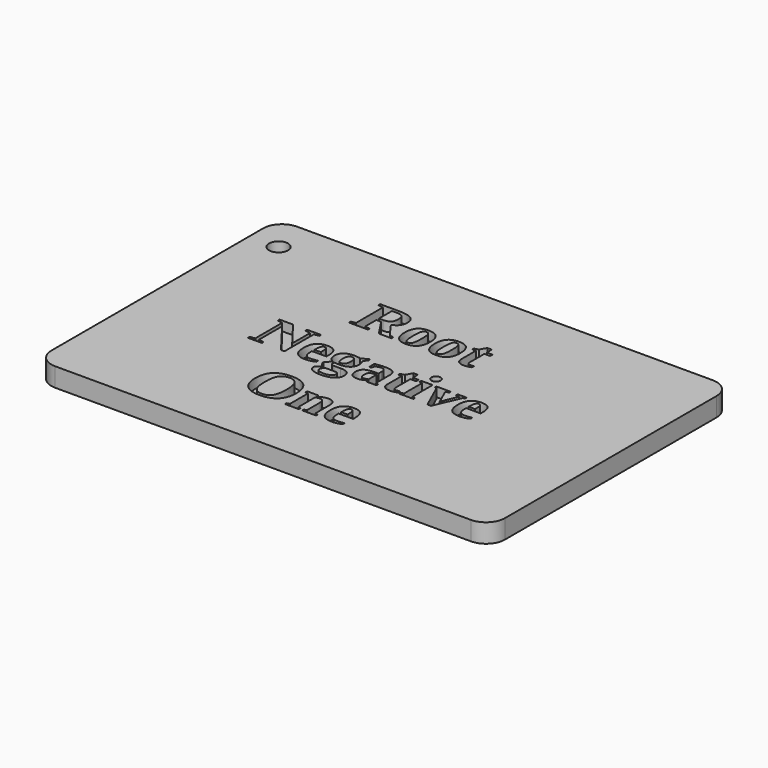
from build123d import *

# Parameters (mm, degrees)
F1_DEPTH     = 6.35
F2_TEXT_SIZE = 20.280284443
F3_DEPTH     = 3.175
F4_R         = 3.175
F5_DEPTH     = 6.35


# Not quite as in the source:
# - Text() gives the source's letters only with a copy of the font that has no kerning and outlines rounded to 1/6400 em; it was checked with that copy


with BuildPart() as f1:
    # F0 (on Top) → F1 (new body)
    with BuildSketch(Plane.XY):
        with BuildLine():
            Line((72.6131111443, 43.1191008464), (-67.0868888557, 43.1191008464))
            ThreePointArc((-67.0868888557, 43.1191008464), (-71.5770169162, 41.2592289069), (-73.4368888557, 36.7691008464))
            Line((-73.4368888557, 36.7691008464), (-73.4368888557, -52.1308991536))
            ThreePointArc((-73.4368888557, -52.1308991536), (-71.5770169162, -56.6210272142), (-67.0868888557, -58.4808991536))
            Line((-67.0868888557, -58.4808991536), (72.6131111443, -58.4808991536))
            ThreePointArc((72.6131111443, -58.4808991536), (77.1032392048, -56.6210272142), (78.9631111443, -52.1308991536))
            Line((78.9631111443, -52.1308991536), (78.9631111443, 36.7691008464))
            ThreePointArc((78.9631111443, 36.7691008464), (77.1032392048, 41.2592289069), (72.6131111443, 43.1191008464))
        make_face()
    extrude(amount=F1_DEPTH)

    # F2 (on face) → F3 (cut)
    with BuildSketch(Plane.XY.offset(6.35)):
        with Locations((-22.8897866678, 9.0731099481)):
            Text('Root', F2_TEXT_SIZE, font='Tinos', font_style=FontStyle.BOLD, text_align=(TextAlign.LEFT, TextAlign.BOTTOM))
        with Locations((-38.1, -14.2492171613)):
            Text('Negative', F2_TEXT_SIZE, font='Tinos', font_style=FontStyle.BOLD, text_align=(TextAlign.LEFT, TextAlign.BOTTOM))
        with Locations((-22.8897866678, -37.5715442708)):
            Text('One', F2_TEXT_SIZE, font='Tinos', font_style=FontStyle.BOLD, text_align=(TextAlign.LEFT, TextAlign.BOTTOM))
    extrude(amount=-F3_DEPTH, mode=Mode.SUBTRACT)

    # F4 (on face) → F5 (cut)
    with BuildSketch(Plane.XY.offset(6.35)):
        with Locations((-63.6921020849, 31.1142940747)):
            Circle(F4_R)
    extrude(amount=-F5_DEPTH, mode=Mode.SUBTRACT)


solid = f1.part
